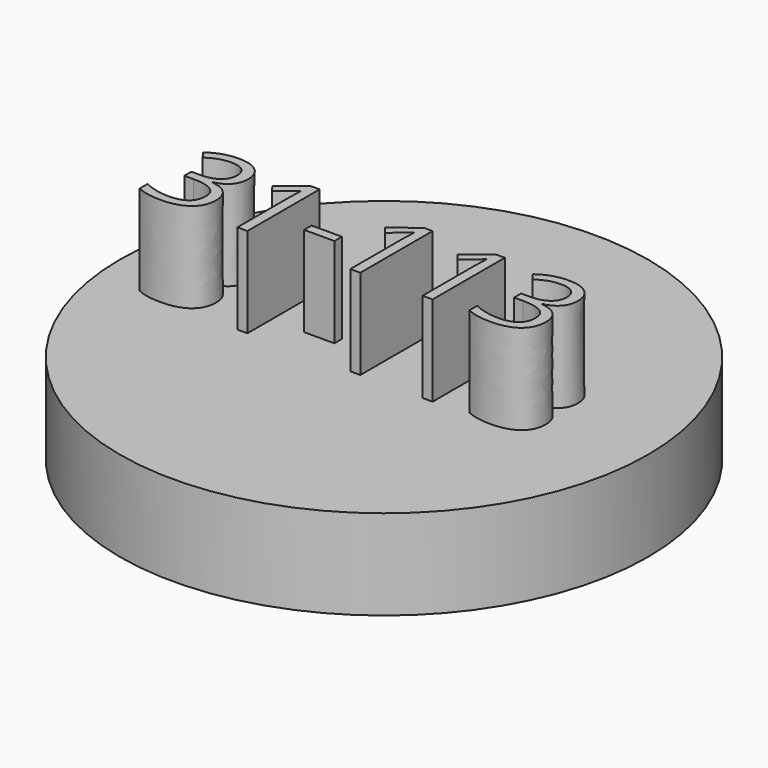
from build123d import *

# Parameters (mm, degrees)
F0_R         = 74.4932059344
F1_DEPTH     = 25.4
F2_TEXT_SIZE = 35.6493336666
F3_DEPTH     = 25.4


# Not quite as in the source:
# - Text() gives the source's letters only with a copy of the font that has no kerning and outlines rounded to 1/6400 em; it was checked with that copy


with BuildPart() as f1:
    # F0 (on Top) → F1 (new body)
    with BuildSketch(Plane.XY):
        Circle(F0_R)
    extrude(amount=F1_DEPTH)

    # F2 (on face) → F3 (join)
    with BuildSketch(Plane.XY.offset(25.4)):
        with Locations((-63.4048879147, -9.9308919162)):
            Text('31-113', F2_TEXT_SIZE, font='Open Sans', text_align=(TextAlign.LEFT, TextAlign.BOTTOM))
    extrude(amount=F3_DEPTH)


solid = f1.part
